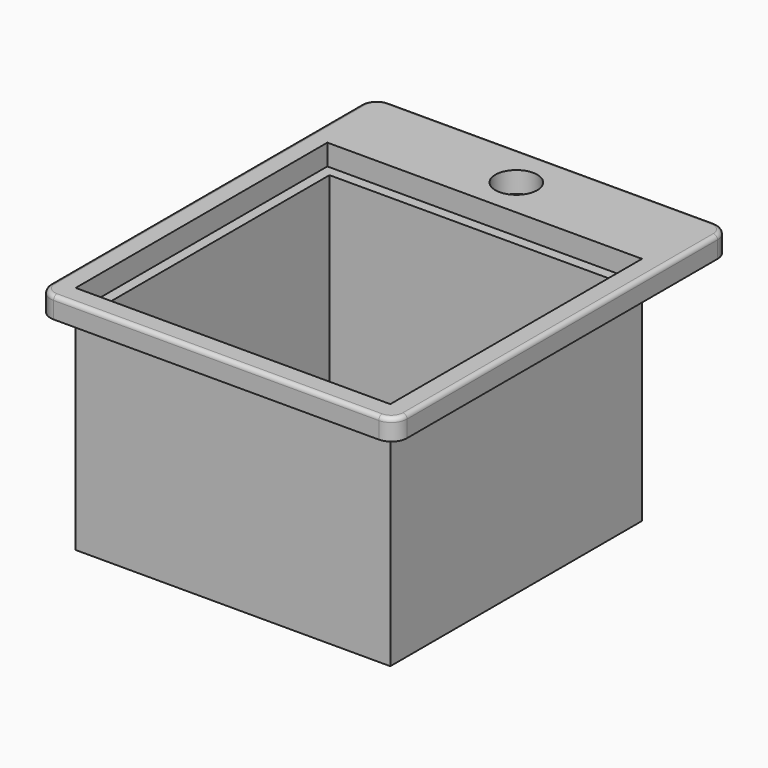
from build123d import *

# Parameters (mm, degrees)
F1_W     = 381
F1_H     = 381
F4_DEPTH = 254
F2_W     = 381
F2_H     = 381
F5_DEPTH = 25.4
F6_R     = 5.08
F7_D     = 50.8
F8_T     = -12.7
F9_D     = 76.2


with BuildPart() as f4:
    # F1 (on Top) → F4 (new body)
    with BuildSketch(Plane.XY):
        Rectangle(F1_W, F1_H)
    extrude(amount=-F4_DEPTH)

    # F8
    f8_openings = [f4.faces().sort_by_distance(p)[0] for p in [
        (0, 0, 0),
    ]]
    offset(amount=F8_T, openings=f8_openings)

    # F9 (through all)
    with Locations(Plane.XY):
        with Locations((0, 0)):
            Hole(F9_D / 2)


with BuildPart() as f5:
    # F2 (on face) → F5 (new body)
    with BuildSketch(Plane.XY):
        with BuildLine():
            Line((196.85, 292.1), (-196.85, 292.1))
            ThreePointArc((-196.85, 292.1), (-210.3203841816, 286.5203841816), (-215.9, 273.05))
            Line((-215.9, 273.05), (-215.9, -196.85))
            ThreePointArc((-215.9, -196.85), (-210.3203841816, -210.3203841816), (-196.85, -215.9))
            Line((-196.85, -215.9), (196.85, -215.9))
            ThreePointArc((196.85, -215.9), (210.3203841816, -210.3203841816), (215.9, -196.85))
            Line((215.9, -196.85), (215.9, 273.05))
            ThreePointArc((215.9, 273.05), (210.3203841816, 286.5203841816), (196.85, 292.1))
        make_face()
        Rectangle(F2_W, F2_H, mode=Mode.SUBTRACT)
    extrude(amount=F5_DEPTH)

    # F6
    f6_edges = [f5.edges().sort_by_distance(p)[0] for p in [
        (-215.9, 38.1, 25.4),
        (-210.320384, 286.520384, 25.4),
        (0, 292.1, 25.4),
        (210.320384, 286.520384, 25.4),
        (215.9, 38.1, 25.4),
        (210.320384, -210.320384, 25.4),
        (0, -215.9, 25.4),
        (-210.320384, -210.320384, 25.4),
    ]]
    fillet(f6_edges, radius=F6_R)

    # F7 (through all)
    with Locations(Plane(origin=(0, 0, 0), x_dir=(1, 0, 0), z_dir=(0, 0, -1))):
        with Locations((0, -238.4229451418)):
            Hole(F7_D / 2)


solid = Compound([f4.part, f5.part])
